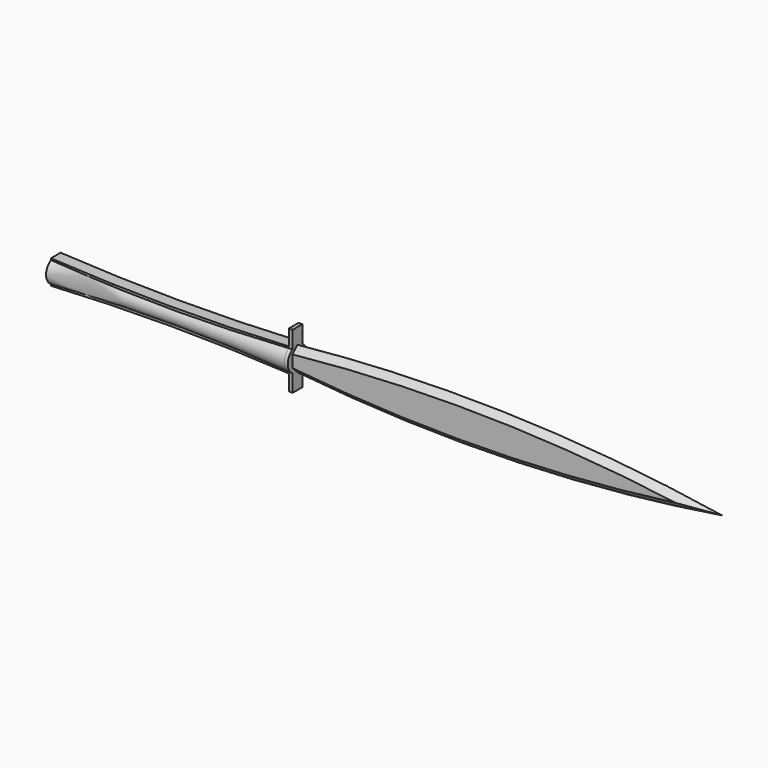
from build123d import *

# Parameters (mm, degrees)
F2_DEPTH     = 0.635
F3_T4_ANGLE  = 16.069160735
F3_S5_R      = 171.2764102712
F3_T6_DEPTH  = 27
F3_T11_ANGLE = 16.069160735
F3_S13_R     = 171.2764102712
F3_T14_DEPTH = 27
F3_T18_ANGLE = 16.069160735
F3_S20_R     = 171.2764102712
F3_T21_DEPTH = 27
F3_T25_ANGLE = 16.069160735
F3_S27_R     = 171.2764102712
F3_T28_DEPTH = 27
F3_T33_ANGLE = 16.069160735
F3_S34_R     = 171.2764102712
F3_T35_DEPTH = 27
F3_T38_ANGLE = 16.069160735
F3_S39_R     = 171.2764102712
F3_T40_DEPTH = 27
F3_T46_ANGLE = 16.069160735
F3_S47_R     = 171.2764102712
F3_T48_DEPTH = 27
F3_T51_ANGLE = 16.069160735
F3_S52_R     = 171.2764102712
F3_T53_DEPTH = 27


# Not quite as in the source:
# - a fillet or chamfer that OpenCascade refuses, or shapes differently, is made with other operations: its cross-section is extruded or revolved along the edge and cut away or added


with BuildPart() as f1:
    # F0 (on Front) → F1 (revolve)
    with BuildSketch(Plane.XZ):
        with BuildLine():
            Line((-25.4078488797, 1.2755064527), (0, 1.2755064527))
            Line((0, 1.2755064527), (0, 2.5510129053))
            ThreePointArc((0, 2.5510129053), (-0.1948502254, 2.5399588642), (-0.3897100687, 2.5290756822))
            ThreePointArc((-0.3897100687, 2.5290756822), (-12.8990879478, 2.1882478839), (-25.4078488797, 2.5510129053))
            Line((-25.4078488797, 2.5510129053), (-25.4078488797, 1.2755064527))
        make_face()
    revolve(axis=Axis((-12.7039244398, 0, 1.2755064527), (1, 0, 0)))

    # F0 (on Front) → F2 (join, symmetric)
    with BuildSketch(Plane.XZ):
        with BuildLine():
            ThreePointArc((-0.3897100687, 0.0219372231), (-0.1948502254, 0.0110540411), (0, 0))
            Line((0, 0), (0, 1.2755064527))
            Line((0, 1.2755064527), (-25.4078488797, 1.2755064527))
            Line((-25.4078488797, 1.2755064527), (-25.4078488797, 0))
            ThreePointArc((-25.4078488797, 0), (-12.8990879478, 0.3627650215), (-0.3897100687, 0.0219372231))
        make_face()
        with BuildLine():
            Line((0, -1.6435489524), (0, 0))
            ThreePointArc((0, 0), (-0.1948502254, 0.0110540411), (-0.3897100687, 0.0219372231))
            Line((-0.3897100687, 0.0219372231), (-0.3897100687, -1.6435489524))
            Line((-0.3897100687, -1.6435489524), (0, -1.6435489524))
        make_face()
        with BuildLine():
            Line((0, 1.2755064527), (0, 0))
            ThreePointArc((0, 0), (22.353983247, -0.8223795413), (44.6244962513, 1.2755064527))
            Line((44.6244962513, 1.2755064527), (0, 1.2755064527))
        make_face()
        with BuildLine():
            Line((-25.4078488797, 1.2755064527), (0, 1.2755064527))
            Line((0, 1.2755064527), (0, 2.5510129053))
            ThreePointArc((0, 2.5510129053), (-0.1948502254, 2.5399588642), (-0.3897100687, 2.5290756822))
            ThreePointArc((-0.3897100687, 2.5290756822), (-12.8990879478, 2.1882478839), (-25.4078488797, 2.5510129053))
            Line((-25.4078488797, 2.5510129053), (-25.4078488797, 1.2755064527))
        make_face()
        with BuildLine():
            Line((0, 2.5510129053), (0, 1.2755064527))
            Line((0, 1.2755064527), (44.6244962513, 1.2755064527))
            ThreePointArc((44.6244962513, 1.2755064527), (22.353983247, 3.3733924466), (0, 2.5510129053))
        make_face()
        with BuildLine():
            ThreePointArc((-0.3897100687, 2.5290756822), (-0.1948502254, 2.5399588642), (0, 2.5510129053))
            Line((0, 2.5510129053), (0, 4.1945618577))
            Line((0, 4.1945618577), (-0.3897100687, 4.1945618577))
            Line((-0.3897100687, 4.1945618577), (-0.3897100687, 2.5290756822))
        make_face()
    extrude(amount=F2_DEPTH, both=True)

    # F3: chamfer of 0.635 on 4 edges, made by hand


with BuildPart() as f3_tool2:
    # F3_s3 → F3_t4 (revolve)
    with BuildSketch(Plane(origin=(44.7635003775, 0, -7.6289121798), x_dir=(0, 1, 0), z_dir=(0.9857862022, 0, -0.1680046534))):
        with BuildLine():
            Line((0.0179605122, 8.7802452438), (-0.6529605122, 8.1093242193))
            Line((-0.6529605122, 8.1093242193), (-0.6656605122, 8.1093242193))
            ThreePointArc((-0.6656605122, 8.1093242193), (-0.6477, 8.4358044754), (-0.6477, 8.7622847316))
            Line((-0.6477, 8.7622847316), (-0.635, 8.7749847316))
            ThreePointArc((-0.635, 8.7749847316), (-0.3085197439, 8.7749847316), (0.0179605122, 8.7929452438))
            Line((0.0179605122, 8.7929452438), (0.0179605122, 8.7802452438))
        make_face()
    revolve(axis=Axis((17.4603710483, -0.635, -167.8330947992), (0, -1, 0)), revolution_arc=F3_T4_ANGLE)

    # F3_s5 → F3_t6 (intersect, symmetric)
    with BuildSketch(Plane.XZ.offset(0.5)):
        with Locations((17.4603710483, 170.3841077045)):
            Circle(F3_S5_R)
    extrude(amount=F3_T6_DEPTH, both=True, mode=Mode.INTERSECT)

    split(bisect_by=Plane.YZ, keep=Keep.TOP)


with BuildPart() as f1_1:
    add(f1.part)

    # F3_t1: cut F3_tool2
    add(f3_tool2.part, mode=Mode.SUBTRACT)


with BuildPart() as f3_tool9:
    # F3_s10 → F3_t11 (revolve)
    with BuildSketch(Plane(origin=(44.7635003775, 0, -7.6289121798), x_dir=(0, 1, 0), z_dir=(0.9857862022, 0, -0.1680046534))):
        with BuildLine():
            Line((0.6529605122, 8.1093242193), (-0.0179605122, 8.7802452438))
            Line((-0.0179605122, 8.7802452438), (-0.0179605122, 8.7929452438))
            ThreePointArc((-0.0179605122, 8.7929452438), (0.3085197439, 8.7749847316), (0.635, 8.7749847316))
            Line((0.635, 8.7749847316), (0.6477, 8.7622847316))
            ThreePointArc((0.6477, 8.7622847316), (0.6477, 8.4358044754), (0.6656605122, 8.1093242193))
            Line((0.6656605122, 8.1093242193), (0.6529605122, 8.1093242193))
        make_face()
    revolve(axis=Axis((17.4603710483, 0.635, -167.8330947992), (0, -1, 0)), revolution_arc=F3_T11_ANGLE)

    split(bisect_by=Plane.YZ, keep=Keep.TOP)

    # F3_s13 → F3_t14 (intersect, symmetric)
    with BuildSketch(Plane.XZ.offset(-0.5)):
        with Locations((17.4603710483, 170.3841077045)):
            Circle(F3_S13_R)
    extrude(amount=F3_T14_DEPTH, both=True, mode=Mode.INTERSECT)


with BuildPart() as f1_2:
    add(f1_1.part)

    # F3_t8: cut F3_tool9
    add(f3_tool9.part, mode=Mode.SUBTRACT)


with BuildPart() as f3_tool16:
    # F3_s17 → F3_t18 (revolve)
    with BuildSketch(Plane(origin=(-1.6228435165, 0, 0.1819546373), x_dir=(0, 1, 0), z_dir=(-0.9937731026, 0, 0.1114227112))):
        with BuildLine():
            Line((0.6529605122, -0.6451754671), (-0.0179605122, 0.0257455574))
            Line((-0.0179605122, 0.0257455574), (-0.0179605122, 0.0384455574))
            ThreePointArc((-0.0179605122, 0.0384455574), (0.3085197439, 0.0204850452), (0.635, 0.0204850452))
            Line((0.635, 0.0204850452), (0.6477, 0.0077850452))
            ThreePointArc((0.6477, 0.0077850452), (0.6477, -0.318695211), (0.6656605122, -0.6451754671))
            Line((0.6656605122, -0.6451754671), (0.6529605122, -0.6451754671))
        make_face()
    revolve(axis=Axis((17.4603710483, 0.635, 170.3841077045), (0, -1, 0)), revolution_arc=F3_T18_ANGLE)

    split(bisect_by=Plane.YZ, keep=Keep.TOP)

    # F3_s20 → F3_t21 (intersect, symmetric)
    with BuildSketch(Plane.XZ.offset(-0.5)):
        with Locations((17.4603710483, -167.8330947992)):
            Circle(F3_S20_R)
    extrude(amount=F3_T21_DEPTH, both=True, mode=Mode.INTERSECT)


with BuildPart() as f1_3:
    add(f1_2.part)

    # F3_t15: cut F3_tool16
    add(f3_tool16.part, mode=Mode.SUBTRACT)


with BuildPart() as f3_tool23:
    # F3_s24 → F3_t25 (revolve)
    with BuildSketch(Plane(origin=(-1.6228435165, 0, 0.1819546373), x_dir=(0, 1, 0), z_dir=(-0.9937731026, 0, 0.1114227112))):
        with BuildLine():
            Line((0.0179605122, 0.0257455574), (-0.6529605122, -0.6451754671))
            Line((-0.6529605122, -0.6451754671), (-0.6656605122, -0.6451754671))
            ThreePointArc((-0.6656605122, -0.6451754671), (-0.6477, -0.318695211), (-0.6477, 0.0077850452))
            Line((-0.6477, 0.0077850452), (-0.635, 0.0204850452))
            ThreePointArc((-0.635, 0.0204850452), (-0.3085197439, 0.0204850452), (0.0179605122, 0.0384455574))
            Line((0.0179605122, 0.0384455574), (0.0179605122, 0.0257455574))
        make_face()
    revolve(axis=Axis((17.4603710483, -0.635, 170.3841077045), (0, -1, 0)), revolution_arc=F3_T25_ANGLE)

    split(bisect_by=Plane.YZ, keep=Keep.TOP)

    # F3_s27 → F3_t28 (intersect, symmetric)
    with BuildSketch(Plane.XZ.offset(0.5)):
        with Locations((17.4603710483, -167.8330947992)):
            Circle(F3_S27_R)
    extrude(amount=F3_T28_DEPTH, both=True, mode=Mode.INTERSECT)


with BuildPart() as f1_4:
    add(f1_3.part)

    # F3_t22: cut F3_tool23
    add(f3_tool23.part, mode=Mode.SUBTRACT)


with BuildPart() as f3_tool31:
    # F3_s32 → F3_t33 (revolve)
    with BuildSketch(Plane(origin=(-1.6228435165, 0, 0.1819546373), x_dir=(0, 1, 0), z_dir=(-0.9937731026, 0, 0.1114227112))):
        with BuildLine():
            Line((0.0179605122, 0.0257455574), (-0.6529605122, -0.6451754671))
            Line((-0.6529605122, -0.6451754671), (-0.6656605122, -0.6451754671))
            ThreePointArc((-0.6656605122, -0.6451754671), (-0.6477, -0.318695211), (-0.6477, 0.0077850452))
            Line((-0.6477, 0.0077850452), (-0.635, 0.0204850452))
            ThreePointArc((-0.635, 0.0204850452), (-0.3085197439, 0.0204850452), (0.0179605122, 0.0384455574))
            Line((0.0179605122, 0.0384455574), (0.0179605122, 0.0257455574))
        make_face()
    revolve(axis=Axis((17.4603710483, -0.635, 170.3841077045), (0, -1, 0)), revolution_arc=F3_T33_ANGLE)

    # F3_s34 → F3_t35 (cut, symmetric)
    with BuildSketch(Plane.XZ.offset(0.5)):
        with Locations((17.4603710483, -167.8330947992)):
            Circle(F3_S34_R)
    extrude(amount=F3_T35_DEPTH, both=True, mode=Mode.SUBTRACT)


with BuildPart() as f3_tool36:
    # F3_s37 → F3_t38 (revolve)
    with BuildSketch(Plane(origin=(44.7635003775, 0, -7.6289121798), x_dir=(0, 1, 0), z_dir=(0.9857862022, 0, -0.1680046534))):
        with BuildLine():
            Line((0.0179605122, 8.7802452438), (-0.6529605122, 8.1093242193))
            Line((-0.6529605122, 8.1093242193), (-0.6656605122, 8.1093242193))
            ThreePointArc((-0.6656605122, 8.1093242193), (-0.6477, 8.4358044754), (-0.6477, 8.7622847316))
            Line((-0.6477, 8.7622847316), (-0.635, 8.7749847316))
            ThreePointArc((-0.635, 8.7749847316), (-0.3085197439, 8.7749847316), (0.0179605122, 8.7929452438))
            Line((0.0179605122, 8.7929452438), (0.0179605122, 8.7802452438))
        make_face()
    revolve(axis=Axis((17.4603710483, -0.635, -167.8330947992), (0, -1, 0)), revolution_arc=F3_T38_ANGLE)

    # F3_s39 → F3_t40 (cut, symmetric)
    with BuildSketch(Plane.XZ.offset(0.5)):
        with Locations((17.4603710483, 170.3841077045)):
            Circle(F3_S39_R)
    extrude(amount=F3_T40_DEPTH, both=True, mode=Mode.SUBTRACT)


with BuildPart() as f3_tool31_1:
    add(f3_tool31.part)

    # F3_t41: intersect F3_tool36
    add(f3_tool36.part, mode=Mode.INTERSECT)


with BuildPart() as f1_5:
    add(f1_4.part)

    # F3_t29: cut F3_tool31
    add(f3_tool31_1.part, mode=Mode.SUBTRACT)


with BuildPart() as f3_tool44:
    # F3_s45 → F3_t46 (revolve)
    with BuildSketch(Plane(origin=(44.7635003775, 0, -7.6289121798), x_dir=(0, 1, 0), z_dir=(0.9857862022, 0, -0.1680046534))):
        with BuildLine():
            Line((0.6529605122, 8.1093242193), (-0.0179605122, 8.7802452438))
            Line((-0.0179605122, 8.7802452438), (-0.0179605122, 8.7929452438))
            ThreePointArc((-0.0179605122, 8.7929452438), (0.3085197439, 8.7749847316), (0.635, 8.7749847316))
            Line((0.635, 8.7749847316), (0.6477, 8.7622847316))
            ThreePointArc((0.6477, 8.7622847316), (0.6477, 8.4358044754), (0.6656605122, 8.1093242193))
            Line((0.6656605122, 8.1093242193), (0.6529605122, 8.1093242193))
        make_face()
    revolve(axis=Axis((17.4603710483, 0.635, -167.8330947992), (0, -1, 0)), revolution_arc=F3_T46_ANGLE)

    # F3_s47 → F3_t48 (cut, symmetric)
    with BuildSketch(Plane.XZ.offset(-0.5)):
        with Locations((17.4603710483, 170.3841077045)):
            Circle(F3_S47_R)
    extrude(amount=F3_T48_DEPTH, both=True, mode=Mode.SUBTRACT)


with BuildPart() as f3_tool49:
    # F3_s50 → F3_t51 (revolve)
    with BuildSketch(Plane(origin=(-1.6228435165, 0, 0.1819546373), x_dir=(0, 1, 0), z_dir=(-0.9937731026, 0, 0.1114227112))):
        with BuildLine():
            Line((0.6529605122, -0.6451754671), (-0.0179605122, 0.0257455574))
            Line((-0.0179605122, 0.0257455574), (-0.0179605122, 0.0384455574))
            ThreePointArc((-0.0179605122, 0.0384455574), (0.3085197439, 0.0204850452), (0.635, 0.0204850452))
            Line((0.635, 0.0204850452), (0.6477, 0.0077850452))
            ThreePointArc((0.6477, 0.0077850452), (0.6477, -0.318695211), (0.6656605122, -0.6451754671))
            Line((0.6656605122, -0.6451754671), (0.6529605122, -0.6451754671))
        make_face()
    revolve(axis=Axis((17.4603710483, 0.635, 170.3841077045), (0, -1, 0)), revolution_arc=F3_T51_ANGLE)

    # F3_s52 → F3_t53 (cut, symmetric)
    with BuildSketch(Plane.XZ.offset(-0.5)):
        with Locations((17.4603710483, -167.8330947992)):
            Circle(F3_S52_R)
    extrude(amount=F3_T53_DEPTH, both=True, mode=Mode.SUBTRACT)


with BuildPart() as f3_tool44_1:
    add(f3_tool44.part)

    # F3_t54: intersect F3_tool49
    add(f3_tool49.part, mode=Mode.INTERSECT)


with BuildPart() as f1_6:
    add(f1_5.part)

    # F3_t42: cut F3_tool44
    add(f3_tool44_1.part, mode=Mode.SUBTRACT)


solid = f1_6.part
